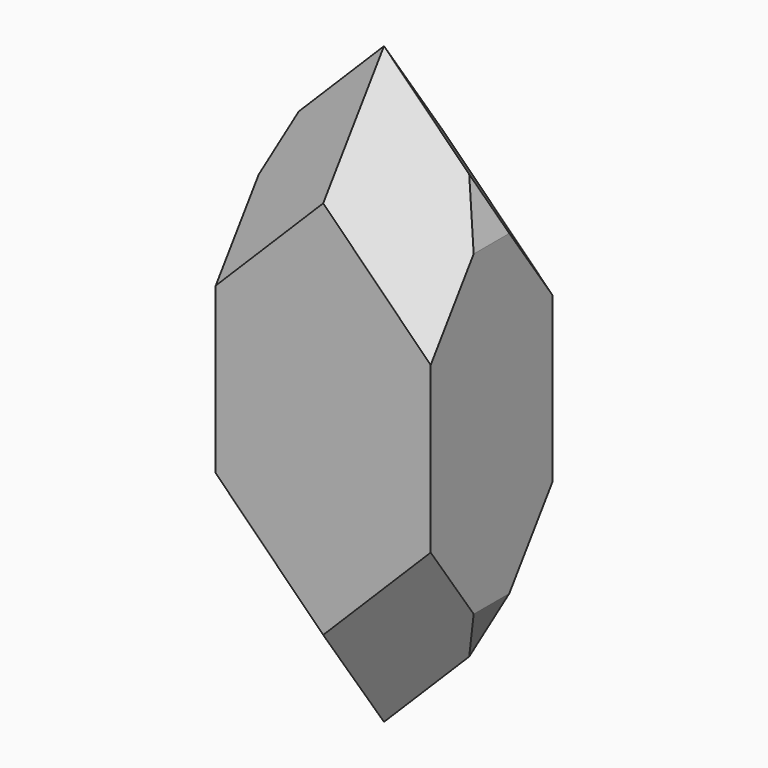
from build123d import *

# Parameters (mm, degrees)
F1_DEPTH    = 5.08
F2_T1_DEPTH = 18.1441495789
F2_T3_DEPTH = 18.1441495789
F2_T5_DEPTH = 18.1441495789
F2_T7_DEPTH = 18.1441495789
F2_T9_DEPTH = 10.8131399699


# Not quite as in the source:
# - a fillet or chamfer that OpenCascade refuses, or shapes differently, is made with other operations: its cross-section is extruded or revolved along the edge and cut away or added


with BuildPart() as f1:
    # F0 (on Front) → F1 (new body)
    with BuildSketch(Plane.XZ):
        Polygon((-25.7146830065, 3.5921024484), (-22.1225805581, 0), (-18.5304781096, 3.5921024484), (-18.5304781096, 16.2921024484), (-22.1225805581, 19.8842048969), (-25.7146830065, 16.2921024484), align=None)
    extrude(amount=F1_DEPTH)

    # F2: chamfer of 2.54 on 12 edges, made by hand

    # F2_s2 → F2_t1 (cut)
    with BuildSketch(Plane(origin=(-12.7924159002, 0, 12.7924159002), x_dir=(0, 1, 0), z_dir=(-0.7071067812, 0, 0.7071067812))):
        Polygon((-2.54, 1.5827706089), (-5.08, 4.1227706089), (-5.08, 1.5827706089), align=None)
        Polygon((-2.54, 1.5827706089), (0, 4.1227706089), (0, 1.5827706089), align=None)
    extrude(amount=F2_T1_DEPTH, mode=Mode.SUBTRACT)

    # F2_s4 → F2_t3 (cut)
    with BuildSketch(Plane(origin=(3.4996865482, 0, 3.4996865482), x_dir=(0, 1, 0), z_dir=(-0.7071067812, 0, -0.7071067812))):
        Polygon((-2.54, -29.703282851), (-5.08, -27.163282851), (-5.08, -29.703282851), align=None)
        Polygon((-2.54, -29.703282851), (0, -27.163282851), (0, -29.703282851), align=None)
    extrude(amount=F2_T3_DEPTH, mode=Mode.SUBTRACT)

    # F2_s6 → F2_t5 (cut)
    with BuildSketch(Plane(origin=(-19.2722671063, 0, 19.2722671063), x_dir=(0, 1, 0), z_dir=(0.7071067812, 0, -0.7071067812))):
        Polygon((-2.54, -15.64302673), (-5.08, -13.10302673), (-5.08, -15.64302673), align=None)
        Polygon((-2.54, -15.64302673), (0, -13.10302673), (0, -15.64302673), align=None)
    extrude(amount=F2_T5_DEPTH, mode=Mode.SUBTRACT)

    # F2_s8 → F2_t7 (cut)
    with BuildSketch(Plane(origin=(-15.6801646579, 0, -15.6801646579), x_dir=(0, 1, 0), z_dir=(0.7071067812, 0, 0.7071067812))):
        Polygon((-2.54, 15.64302673), (-5.08, 18.18302673), (-5.08, 15.64302673), align=None)
        Polygon((-2.54, 15.64302673), (0, 18.18302673), (0, 15.64302673), align=None)
    extrude(amount=F2_T7_DEPTH, mode=Mode.SUBTRACT)

    # F2_s10 → F2_t9 (cut)
    with BuildSketch(Plane.XZ.offset(-2.8665699849)):
        Polygon((-19.2744268854, 2.8481536726), (-18.5304781096, 4.6442048969), (-18.5304781096, 3.5921024484), align=None)
        Polygon((-18.5304781096, 15.24), (-19.2744268854, 17.0360512242), (-18.5304781096, 16.2921024484), align=None)
        Polygon((-25.7146830065, 15.24), (-24.9707342307, 17.0360512242), (-25.7146830065, 16.2921024484), align=None)
        Polygon((-25.7146830065, 4.6442048969), (-24.9707342307, 2.8481536726), (-25.7146830065, 3.5921024484), align=None)
    extrude(amount=F2_T9_DEPTH, mode=Mode.SUBTRACT)


solid = f1.part
